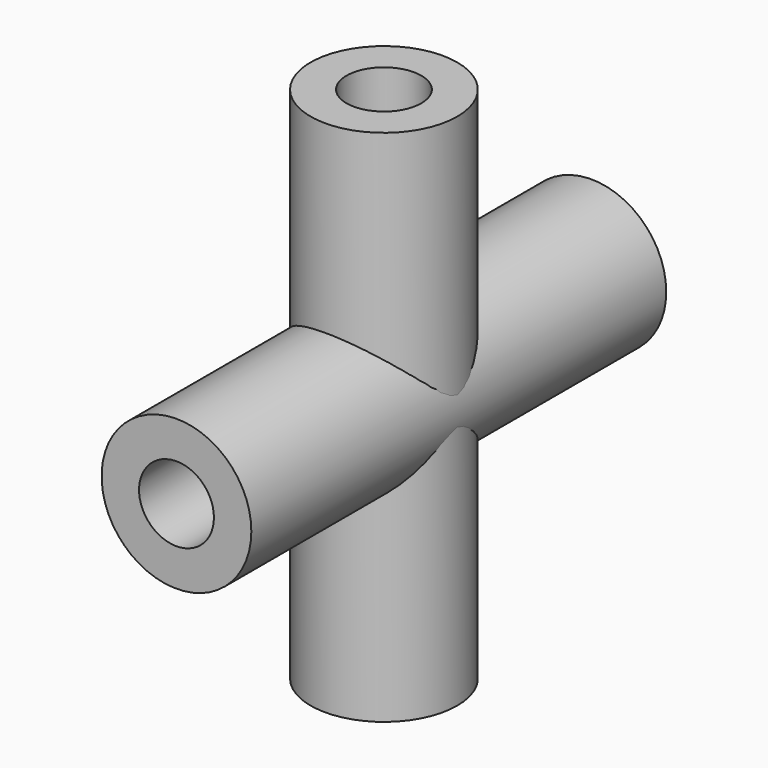
from build123d import *

# Parameters (mm, degrees)
F0_R          = 2.45
F1_DEPTH      = 17.321
F2_R          = 1.25
F3_DEPTH      = 6
F4_R          = 2.5
F5_DEPTH      = 8.6605
F5_DEPTH_BACK = 8.6605
F6_R          = 1.25
F7_DEPTH      = 6
F8_R          = 1.25
F9_DEPTH      = 6
F10_R         = 1.25
F11_DEPTH     = 6


# Not quite as in the source:
# - a feature names something its author has since deleted; it is built from what else it names


with BuildPart() as f1:
    # F0 (on Top) → F1 (new body)
    with BuildSketch(Plane.XY):
        Circle(F0_R)
    extrude(amount=F1_DEPTH)

    # F2 (on face) → F3 (cut)
    with BuildSketch(Plane.XY.offset(17.321)):
        Circle(F2_R)
    extrude(amount=-F3_DEPTH, mode=Mode.SUBTRACT)

    # F6 (on face) → F7 (cut)
    with BuildSketch(Plane(origin=(0, 0, 0), x_dir=(1, 0, 0), z_dir=(0, 0, -1))):
        Circle(F6_R)
    extrude(amount=-F7_DEPTH, mode=Mode.SUBTRACT)


with BuildPart() as f5:
    # F4 (on Front) → F5 (new body, two sides)
    with BuildSketch(Plane.XZ) as f5_sk:
        with Locations((0, 8.6605)):
            Circle(F4_R)
    extrude(amount=F5_DEPTH)
    extrude(f5_sk.sketch, amount=-F5_DEPTH_BACK)

    # F8 (on face) → F9 (cut)
    with BuildSketch(Plane.XZ.offset(8.6605)):
        with Locations((0, 8.6605)):
            Circle(F8_R)
    extrude(amount=-F9_DEPTH, mode=Mode.SUBTRACT)

    # F10 (on face) → F11 (cut)
    with BuildSketch(Plane(origin=(0, 8.6605, 0), x_dir=(-1, 0, 0), z_dir=(0, 1, 0))):
        with Locations((0, 8.6605)):
            Circle(F10_R)
    extrude(amount=-F11_DEPTH, mode=Mode.SUBTRACT)


solid = Compound([f1.part, f5.part])
